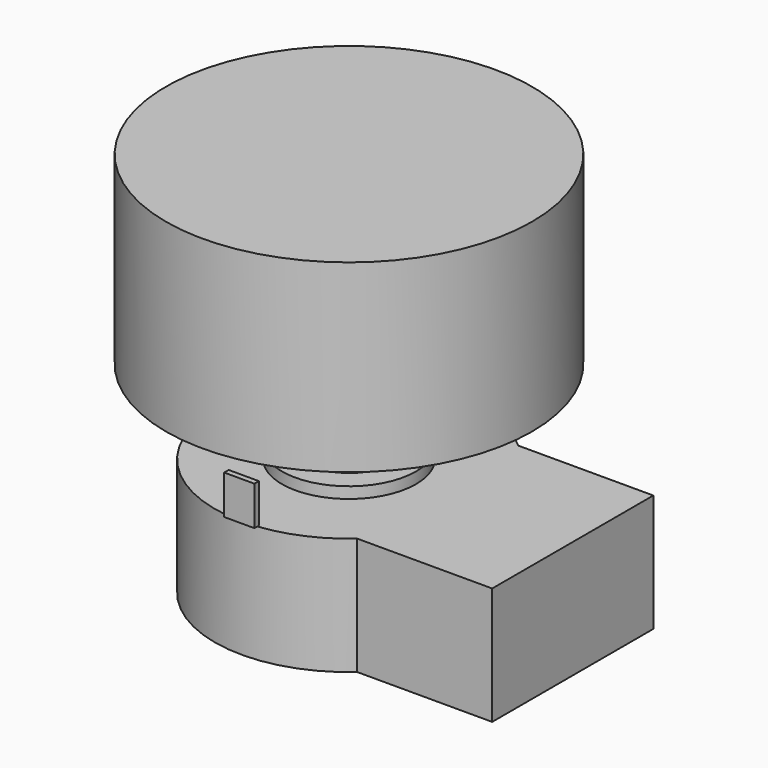
from build123d import *

# Parameters (mm, degrees)
F0_R      = 6
F1_DEPTH  = 1
F2_R      = 12
F2_R_2    = 6
F3_DEPTH  = 10.5
F5_DEPTH  = 10.5
F6_R      = 4
F7_DEPTH  = 6.5
F8_R      = 3
F9_DEPTH  = 8.382
F10_W     = 2.7
F10_H     = 0.5
F11_DEPTH = 3.5
F12_R     = 16.3576
F13_DEPTH = 16.51


with BuildPart() as f1:
    # F0 (on Top) → F1 (new body)
    with BuildSketch(Plane.XY):
        Circle(F0_R)
    extrude(amount=-F1_DEPTH)

    # F2 (on face) → F3 (join)
    with BuildSketch(Plane(origin=(0, 0, -1), x_dir=(1, 0, 0), z_dir=(0, 0, -1))):
        Circle(F2_R)
        Circle(F2_R_2, mode=Mode.SUBTRACT)
        Circle(F2_R_2)
    extrude(amount=F3_DEPTH)

    # F4 (on face) → F5 (join, through all)
    with BuildSketch(Plane.XY.offset(-1)):
        with BuildLine():
            Line((6.35, 9), (6.35, -9))
            Line((6.35, -9), (7.9372539332, -9))
            ThreePointArc((7.9372539332, -9), (10.9372539332, -4.9372539332), (12, 0))
            ThreePointArc((12, 0), (10.9372539332, 4.9372539332), (7.9372539332, 9))
            Line((7.9372539332, 9), (6.35, 9))
        make_face()
        with BuildLine():
            ThreePointArc((12, 0), (10.9372539332, -4.9372539332), (7.9372539332, -9))
            Line((7.9372539332, -9), (20, -9))
            Line((20, -9), (20, 9))
            Line((20, 9), (7.9372539332, 9))
            ThreePointArc((7.9372539332, 9), (10.9372539332, 4.9372539332), (12, 0))
        make_face()
    extrude(amount=-F5_DEPTH)

    # F6 (on face) → F7 (join)
    with BuildSketch(Plane.XY):
        Circle(F6_R)
    extrude(amount=F7_DEPTH)

    # F8 (on face) → F9 (join)
    with BuildSketch(Plane.XY.offset(6.5)):
        Circle(F8_R)
    extrude(amount=F9_DEPTH)

    # F10 (on face) → F11 (join)
    with BuildSketch(Plane.XY.offset(-1)):
        with Locations((0, -12)):
            Rectangle(F10_W, F10_H)
    extrude(amount=F11_DEPTH)

    # F12 (on face) → F13 (join)
    with BuildSketch(Plane.XY.offset(6.5)):
        Circle(F12_R)
    extrude(amount=F13_DEPTH)


solid = f1.part
